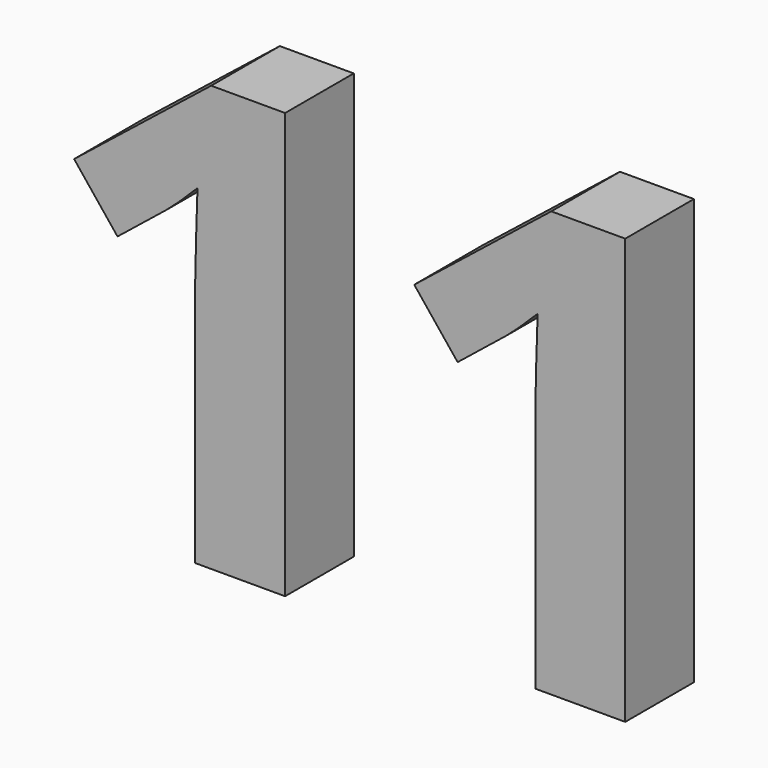
from build123d import *

# Parameters (mm, degrees)
F0_TEXT_SIZE = 35.2777777778
F1_DEPTH     = 5.08


# Not quite as in the source:
# - Text() gives the source's letters only with a copy of the font that has no kerning and outlines rounded to 1/6400 em; it was checked with that copy


with BuildPart() as f1:
    # F0 (on Front) → F1 (new body)
    with BuildSketch(Plane.XZ):
        with Locations((-70.9109674672, 5.6370512024)):
            Text('11', F0_TEXT_SIZE, font='Open Sans', font_style=FontStyle.BOLD, text_align=(TextAlign.LEFT, TextAlign.BOTTOM))
    extrude(amount=F1_DEPTH)


solid = f1.part
